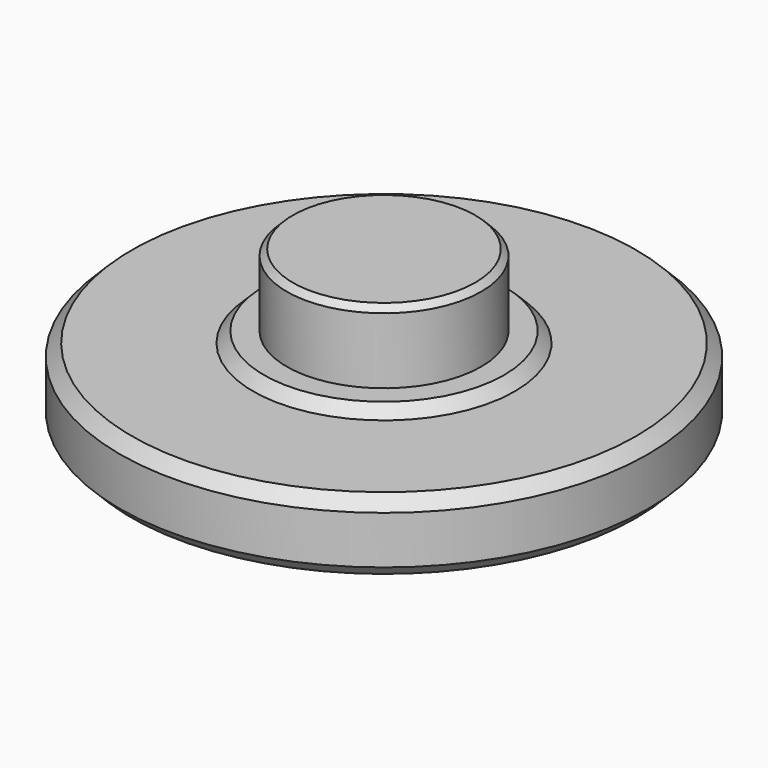
from build123d import *

# Parameters (mm, degrees)
F0_R     = 11
F1_DEPTH = 3
F2_R     = 5.5
F3_DEPTH = 0.45
F4_R     = 4.05
F5_DEPTH = 3
F6_SIZE  = 0.25
F8_SIZE  = 0.5


# Not quite as in the source:
# - a fillet or chamfer that OpenCascade refuses, or shapes differently, is made with other operations: its cross-section is extruded or revolved along the edge and cut away or added


with BuildPart() as f1:
    # F0 (on Top) → F1 (new body)
    with BuildSketch(Plane.XY):
        Circle(F0_R)
    extrude(amount=F1_DEPTH)

    # F2 (on face) → F3 (join)
    with BuildSketch(Plane.XY.offset(3)):
        Circle(F2_R)
    extrude(amount=F3_DEPTH)

    # F4 (on face) → F5 (join)
    with BuildSketch(Plane.XY.offset(3.45)):
        Circle(F4_R)
    extrude(amount=F5_DEPTH)

    # F6
    f6_edges = [f1.edges().sort_by_distance(p)[0] for p in [
        (-4.05, 0, 6.45),
    ]]
    chamfer(f6_edges, length=F6_SIZE)

    # F7: chamfer of 0.5 on 1 edges, made by hand


with BuildPart() as f7_tool2:
    # F7_s3 → F7_t4 (revolve)
    with BuildSketch(Plane.XZ):
        Polygon((5, 3.45), (5.5, 2.95), (5.5, 3.45), align=None)
    revolve(axis=Axis((0, 0, 3.45), (0, 0, 1)))

    split(bisect_by=Plane.XY.offset(3), keep=Keep.TOP)


with BuildPart() as f1_1:
    add(f1.part)

    # F7_t1: cut F7_tool2
    add(f7_tool2.part, mode=Mode.SUBTRACT)

    # F8
    f8_edges = [f1_1.edges().sort_by_distance(p)[0] for p in [
        (-11, 0, 0),
        (-11, 0, 3),
    ]]
    chamfer(f8_edges, length=F8_SIZE)


solid = f1_1.part
